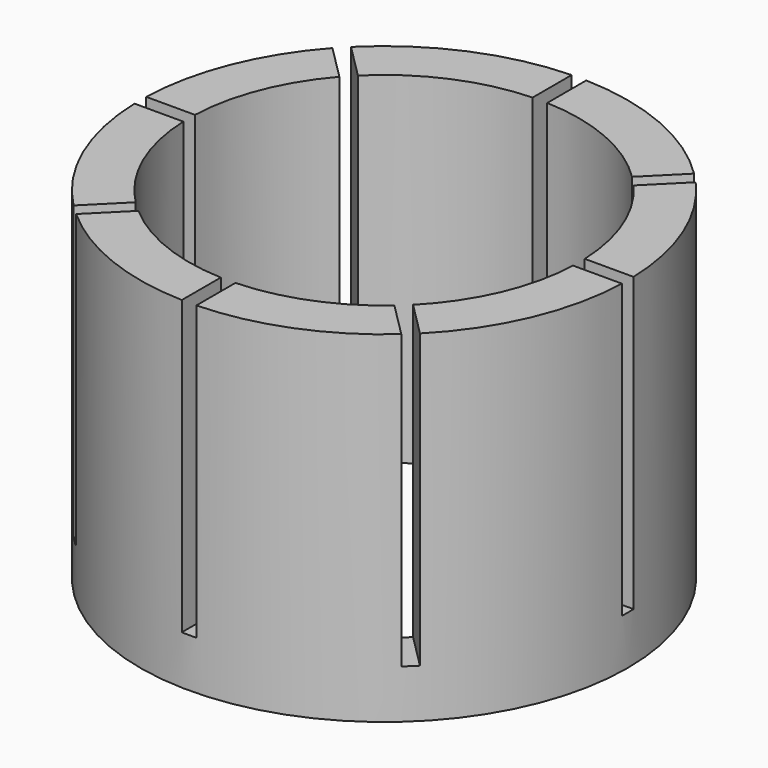
from build123d import *

# Parameters (mm, degrees)
F0_R     = 63.5
F0_R_2   = 50.8
F1_DEPTH = 88.9
F4_DEPTH = 76.2


# Not quite as in the source:
# - a feature of the source that left no trace in its solid (it failed there, or was rolled back) is left out


with BuildPart() as f1:
    # F0 (on Top) → F1 (new body)
    with BuildSketch(Plane.XY):
        Circle(F0_R)
        Circle(F0_R_2, mode=Mode.SUBTRACT)
    extrude(amount=F1_DEPTH)

    # F3 (on face) → F4 (cut)
    with BuildSketch(Plane.XY.offset(88.9)):
        with BuildLine():
            Line((-1.905, -6.8671500075), (-1.905, -3.0571500075))
            Line((-1.905, -3.0571500075), (-2.6940768363, -2.2680731712))
            Line((-2.6940768363, -2.2680731712), (-36.1333947901, -35.7073911249))
            ThreePointArc((-36.1333947901, -35.7073911249), (-34.768258257, -37.0379294477), (-33.3541627773, -38.3163127848))
            Line((-33.3541627773, -38.3163127848), (-1.905, -6.8671500075))
        make_face()
        with BuildLine():
            ThreePointArc((-45.1137772181, -44.6877735529), (-43.7523970967, -46.0214922432), (-42.3516057863, -47.3137557938))
            Line((-42.3516057863, -47.3137557938), (-33.3541627773, -38.3163127848))
            ThreePointArc((-33.3541627773, -38.3163127848), (-34.768258257, -37.0379294477), (-36.1333947901, -35.7073911249))
            Line((-36.1333947901, -35.7073911249), (-45.1137772181, -44.6877735529))
        make_face()
        with BuildLine():
            Line((-44.6998995402, -49.6620495477), (-42.3516057863, -47.3137557938))
            ThreePointArc((-42.3516057863, -47.3137557938), (-43.7523970967, -46.0214922432), (-45.1137772181, -44.6877735529))
            Line((-45.1137772181, -44.6877735529), (-47.3939763765, -46.9679727114))
            Line((-47.3939763765, -46.9679727114), (-44.6998995402, -49.6620495477))
        make_face()
        with BuildLine():
            Line((-67.31, -1.905), (-63.4714185677, -1.905))
            ThreePointArc((-63.4714185677, -1.905), (-63.5, 0), (-63.4714185677, 1.905))
            Line((-63.4714185677, 1.905), (-67.31, 1.905))
            Line((-67.31, 1.905), (-67.31, -1.905))
        make_face()
        with BuildLine():
            ThreePointArc((-63.4714185677, 1.905), (-63.5, 0), (-63.4714185677, -1.905))
            Line((-63.4714185677, -1.905), (-50.7642686838, -1.905))
            ThreePointArc((-50.7642686838, -1.905), (-50.8, 0), (-50.7642686838, 1.905))
            Line((-50.7642686838, 1.905), (-63.4714185677, 1.905))
        make_face()
        with BuildLine():
            Line((-50.7642686838, -1.905), (-3.0571500075, -1.905))
            Line((-3.0571500075, -1.905), (-6.8671500075, 1.905))
            Line((-6.8671500075, 1.905), (-50.7642686838, 1.905))
            ThreePointArc((-50.7642686838, 1.905), (-50.8, 0), (-50.7642686838, -1.905))
        make_face()
        with BuildLine():
            Line((-6.8671500075, 1.905), (-1.905, 1.905))
            Line((-1.905, 1.905), (-1.905, 2.3310036652))
            Line((-1.905, 2.3310036652), (-35.7073911249, 36.1333947901))
            ThreePointArc((-35.7073911249, 36.1333947901), (-37.0379294477, 34.768258257), (-38.3163127848, 33.3541627773))
            Line((-38.3163127848, 33.3541627773), (-6.8671500075, 1.905))
        make_face()
        with BuildLine():
            Line((1.905, 1.905), (6.8671500075, 1.905))
            Line((6.8671500075, 1.905), (38.3163127848, 33.3541627773))
            ThreePointArc((38.3163127848, 33.3541627773), (37.0379294477, 34.768258257), (35.7073911249, 36.1333947901))
            Line((35.7073911249, 36.1333947901), (1.905, 2.3310036652))
            Line((1.905, 2.3310036652), (1.905, 1.905))
        make_face()
        with BuildLine():
            Line((3.0571500075, -1.905), (50.7642686838, -1.905))
            ThreePointArc((50.7642686838, -1.905), (50.7910663854, -0.9526675347), (50.8, 0))
            ThreePointArc((50.8, 0), (50.7910663854, 0.9526675347), (50.7642686838, 1.905))
            Line((50.7642686838, 1.905), (6.8671500075, 1.905))
            Line((6.8671500075, 1.905), (3.0571500075, -1.905))
        make_face()
        with BuildLine():
            Line((50.7642686838, -1.905), (63.4714185677, -1.905))
            ThreePointArc((63.4714185677, -1.905), (63.4928542399, -0.9526071985), (63.5, 0))
            ThreePointArc((63.5, 0), (63.4928542399, 0.9526071985), (63.4714185677, 1.905))
            Line((63.4714185677, 1.905), (50.7642686838, 1.905))
            ThreePointArc((50.7642686838, 1.905), (50.7910663854, 0.9526675347), (50.8, 0))
            ThreePointArc((50.8, 0), (50.7910663854, -0.9526675347), (50.7642686838, -1.905))
        make_face()
        with BuildLine():
            Line((38.3163127848, 33.3541627773), (47.3137557938, 42.3516057863))
            ThreePointArc((47.3137557938, 42.3516057863), (46.0214922432, 43.7523970967), (44.6877735529, 45.1137772181))
            Line((44.6877735529, 45.1137772181), (35.7073911249, 36.1333947901))
            ThreePointArc((35.7073911249, 36.1333947901), (37.0379294477, 34.768258257), (38.3163127848, 33.3541627773))
        make_face()
        with BuildLine():
            ThreePointArc((33.3541627773, -38.3163127848), (34.768258257, -37.0379294477), (36.1333947901, -35.7073911249))
            Line((36.1333947901, -35.7073911249), (2.6940768363, -2.2680731712))
            Line((2.6940768363, -2.2680731712), (1.905, -3.0571500075))
            Line((1.905, -3.0571500075), (1.905, -6.8671500075))
            Line((1.905, -6.8671500075), (33.3541627773, -38.3163127848))
        make_face()
        with BuildLine():
            ThreePointArc((42.3516057863, -47.3137557938), (43.7523970967, -46.0214922432), (45.1137772181, -44.6877735529))
            Line((45.1137772181, -44.6877735529), (36.1333947901, -35.7073911249))
            ThreePointArc((36.1333947901, -35.7073911249), (34.768258257, -37.0379294477), (33.3541627773, -38.3163127848))
            Line((33.3541627773, -38.3163127848), (42.3516057863, -47.3137557938))
        make_face()
        with BuildLine():
            Line((52.015964851, -51.5899611858), (45.1137772181, -44.6877735529))
            ThreePointArc((45.1137772181, -44.6877735529), (43.7523970967, -46.0214922432), (42.3516057863, -47.3137557938))
            Line((42.3516057863, -47.3137557938), (49.3218880147, -54.2840380222))
            Line((49.3218880147, -54.2840380222), (52.015964851, -51.5899611858))
        make_face()
        with BuildLine():
            Line((63.4714185677, -1.905), (67.31, -1.905))
            Line((67.31, -1.905), (67.31, 1.905))
            Line((67.31, 1.905), (63.4714185677, 1.905))
            ThreePointArc((63.4714185677, 1.905), (63.4928542399, 0.9526071985), (63.5, 0))
            ThreePointArc((63.5, 0), (63.4928542399, -0.9526071985), (63.4714185677, -1.905))
        make_face()
        with BuildLine():
            ThreePointArc((44.6877735529, 45.1137772181), (46.0214922432, 43.7523970967), (47.3137557938, 42.3516057863))
            Line((47.3137557938, 42.3516057863), (51.0685980704, 46.106448063))
            Line((51.0685980704, 46.106448063), (48.3745212341, 48.8005248993))
            Line((48.3745212341, 48.8005248993), (44.6877735529, 45.1137772181))
        make_face()
        with BuildLine():
            Line((-35.7073911249, 36.1333947901), (-44.6877735529, 45.1137772181))
            ThreePointArc((-44.6877735529, 45.1137772181), (-46.0214922432, 43.7523970967), (-47.3137557938, 42.3516057863))
            Line((-47.3137557938, 42.3516057863), (-38.3163127848, 33.3541627773))
            ThreePointArc((-38.3163127848, 33.3541627773), (-37.0379294477, 34.768258257), (-35.7073911249, 36.1333947901))
        make_face()
        with BuildLine():
            Line((-1.4789963348, 1.905), (1.4789963348, 1.905))
            Line((1.4789963348, 1.905), (1.905, 2.3310036652))
            Line((1.905, 2.3310036652), (1.905, 50.7642686838))
            ThreePointArc((1.905, 50.7642686838), (0, 50.8), (-1.905, 50.7642686838))
            Line((-1.905, 50.7642686838), (-1.905, 2.3310036652))
            Line((-1.905, 2.3310036652), (-1.4789963348, 1.905))
        make_face()
        with BuildLine():
            Line((1.905, 50.7642686838), (1.905, 63.4714185677))
            ThreePointArc((1.905, 63.4714185677), (0, 63.5), (-1.905, 63.4714185677))
            Line((-1.905, 63.4714185677), (-1.905, 50.7642686838))
            ThreePointArc((-1.905, 50.7642686838), (0, 50.8), (1.905, 50.7642686838))
        make_face()
        with BuildLine():
            ThreePointArc((-47.3137557938, 42.3516057863), (-46.0214922432, 43.7523970967), (-44.6877735529, 45.1137772181))
            Line((-44.6877735529, 45.1137772181), (-47.5721312908, 47.998134956))
            Line((-47.5721312908, 47.998134956), (-50.2662081271, 45.3040581197))
            Line((-50.2662081271, 45.3040581197), (-47.3137557938, 42.3516057863))
        make_face()
        with BuildLine():
            ThreePointArc((-1.905, 63.4714185677), (0, 63.5), (1.905, 63.4714185677))
            Line((1.905, 63.4714185677), (1.905, 67.31))
            Line((1.905, 67.31), (-1.905, 67.31))
            Line((-1.905, 67.31), (-1.905, 63.4714185677))
        make_face()
        with BuildLine():
            ThreePointArc((-1.905, -63.4714185677), (0, -63.5), (1.905, -63.4714185677))
            Line((1.905, -63.4714185677), (1.905, -50.7642686838))
            ThreePointArc((1.905, -50.7642686838), (0, -50.8), (-1.905, -50.7642686838))
            Line((-1.905, -50.7642686838), (-1.905, -63.4714185677))
        make_face()
        with BuildLine():
            Line((1.905, -50.7642686838), (1.905, -6.8671500075))
            Line((1.905, -6.8671500075), (0, -4.9621500075))
            Line((0, -4.9621500075), (-1.905, -6.8671500075))
            Line((-1.905, -6.8671500075), (-1.905, -50.7642686838))
            ThreePointArc((-1.905, -50.7642686838), (0, -50.8), (1.905, -50.7642686838))
        make_face()
    extrude(amount=-F4_DEPTH, mode=Mode.SUBTRACT)


solid = f1.part
